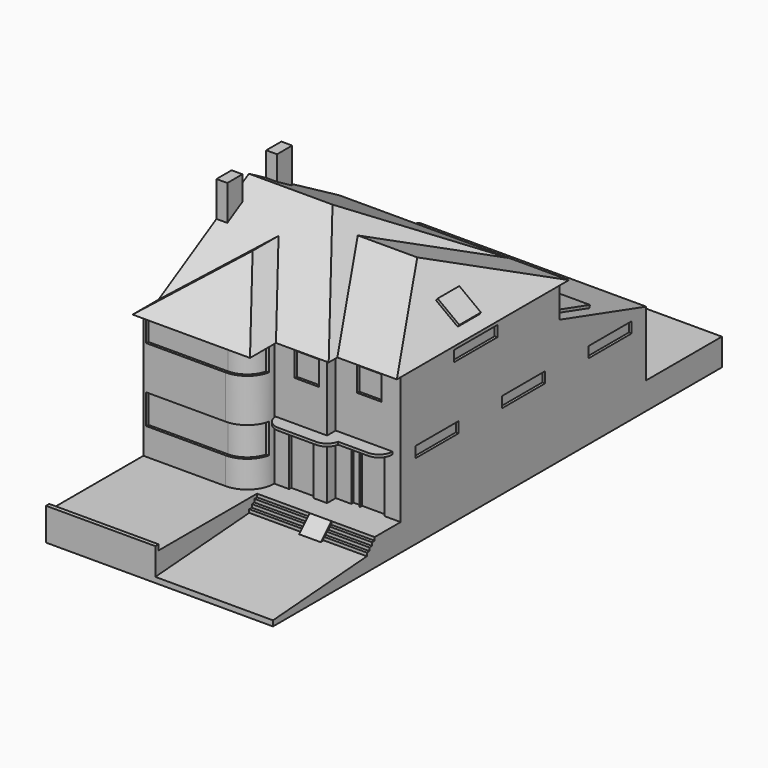
from build123d import *

# Parameters (mm, degrees)
F1_DEPTH  = 4800
F2_W      = 8392
F2_H      = 4000
F3_DEPTH  = 2400
F5_DEPTH  = 8392
F7_DEPTH  = 5992
F8_DEPTH  = 300
F11_DEPTH = 12755.001
F14_DEPTH = 500
F16_DEPTH = 8392.001
F18_DEPTH = 100
F20_DEPTH = 12755.001
F21_W     = 2000
F21_H     = 400
F22_DEPTH = 100
F23_W     = 900
F23_H     = 900
F23_H_2   = 2000
F23_W_2   = 300
F24_DEPTH = 100
F25_W     = 900
F25_H     = 2000
F25_H_2   = 900
F26_DEPTH = 100
F29_DEPTH = 1100
F32_DEPTH = 900
F34_DEPTH = 100
F36_DEPTH = 400
F37_R     = 499.99999
F38_W     = 1900
F38_H     = 2300
F39_DEPTH = 2000
F40_W     = 1238
F40_H     = 2000
F40_H_2   = 1000
F41_DEPTH = 100
F42_W     = 1200
F42_H     = 1484.5474734546
F43_DEPTH = 100
F44_W     = 1000
F44_H     = 1000
F45_DEPTH = 100
F46_W     = 671.4527505016
F46_H     = 900
F46_W_2   = 1200
F47_DEPTH = 100
F48_W     = 8392
F48_H     = 20755
F49_DEPTH = 1000
F51_DEPTH = 4350
F52_W     = 4042
F52_H     = 200
F53_DEPTH = 150
F55_DEPTH = 800


# Not quite as in the source:
# - a fillet or chamfer is up to 0.001 mm smaller than in the source, because OpenCascade refuses the exact size


with BuildPart() as f1:
    # F0 (on Top) → F1 (new body)
    with BuildSketch(Plane.XY):
        with BuildLine():
            Line((0, 11355), (0, -1400))
            Line((0, -1400), (3042, -1400))
            ThreePointArc((3042, -1400), (3749.1067811865, -1107.1067811865), (4042, -400))
            Line((4042, -400), (5992, -400))
            Line((5992, -400), (5992, 0))
            Line((5992, 0), (8392, 0))
            Line((8392, 0), (8392, 11355))
            Line((8392, 11355), (0, 11355))
        make_face()
    extrude(amount=F1_DEPTH)

    # F2 (on face) → F3 (cut)
    with BuildSketch(Plane.XY.offset(4800)):
        with Locations((4196, 9355)):
            Rectangle(F2_W, F2_H)
    extrude(amount=-F3_DEPTH, mode=Mode.SUBTRACT)

    # F4 (on face) → F5 (join, through all)
    with BuildSketch(Plane.YZ.offset(8392)):
        Polygon((7355, 2400), (11355, 2400), (7355, 3600), align=None)
    extrude(amount=-F5_DEPTH)

    # F6 (on face) → F7 (join, through all)
    with BuildSketch(Plane.YZ.offset(5992)):
        Polygon((3477.5, 7200), (-700, 4800), (-400, 4800), (0, 4800), (7655, 4800), align=None)
    extrude(amount=-F7_DEPTH)

    # F6 (on face) → F8 (join)
    with BuildSketch(Plane.YZ.offset(5992)):
        Polygon((3477.5, 7200), (-700, 4800), (7655, 4800), align=None)
    extrude(amount=F8_DEPTH)

    # F10 (on face) → F11 (cut, through all)
    with BuildSketch(Plane.XZ.offset(1400)):
        Polygon((2292, 7800), (6292, 4800), (6292, 7800), align=None)
    extrude(amount=-F11_DEPTH, mode=Mode.SUBTRACT)

    # F12 (on face) → F13 (join, up to the next surface of F1)
    with BuildSketch(Plane.XZ.offset(1400)):
        Polygon((2171, 6428.25), (0, 4800), (3042, 4800), (4342, 4800), align=None)
    extrude(until=Until.NEXT, dir=(0, 1, 0))

    # F12 (on face) → F14 (join)
    with BuildSketch(Plane.XZ.offset(1400)):
        Polygon((2171, 6428.25), (0, 4800), (4342, 4800), align=None)
    extrude(amount=F14_DEPTH)

    # F15 (on face) → F16 (cut, through all)
    with BuildSketch(Plane(origin=(0, 0, 0), x_dir=(0, -1, 0), z_dir=(-1, 0, 0))):
        Polygon((-934.17265625, 6428.25), (1900, 4800), (1900, 6428.25), align=None)
    extrude(amount=-F16_DEPTH, mode=Mode.SUBTRACT)

    # F9 (on face) → F17 (join, up to the next surface of F1)
    with BuildSketch(Plane.YZ.offset(8392)):
        Polygon((3477.5, 6500), (-300, 4800), (0, 4800), (7355, 4800), (7655, 4800), align=None)
    extrude(until=Until.NEXT, dir=(-1, 0, 0))

    # F9 (on face) → F18 (join)
    with BuildSketch(Plane.YZ.offset(8392)):
        Polygon((3477.5, 6500), (-300, 4800), (7655, 4800), align=None)
    extrude(amount=F18_DEPTH)

    # F19 (on face) → F20 (cut, through all)
    with BuildSketch(Plane.XZ.offset(1400)):
        Polygon((6225.3333333333, 6500), (8492, 4800), (8492, 6500), align=None)
    extrude(amount=-F20_DEPTH, mode=Mode.SUBTRACT)

    # F21 (on face) → F22 (cut)
    with BuildSketch(Plane.YZ.offset(8392)):
        with Locations((5677.5, 2000)):
            Rectangle(F21_W, F21_H)
        with Locations((1677.5, 2000)):
            Rectangle(F21_W, F21_H)
        with Locations((3477.5, 4400)):
            Rectangle(F21_W, F21_H)
        with Locations((9677.5, 2000)):
            Rectangle(F21_W, F21_H)
    extrude(amount=-F22_DEPTH, mode=Mode.SUBTRACT)

    # F23 (on face) → F24 (cut)
    with BuildSketch(Plane.XZ):
        with Locations((7233.0629348755, 4134.8165988922)):
            Rectangle(F23_W, F23_H)
        with Locations((7342, 1000)):
            Rectangle(F23_W, F23_H_2)
        with Locations((6722, 1000)):
            Rectangle(F23_W_2, F23_H_2)
    extrude(amount=-F24_DEPTH, mode=Mode.SUBTRACT)

    # F25 (on face) → F26 (cut)
    with BuildSketch(Plane.XZ.offset(400)):
        with Locations((5042, 1000)):
            Rectangle(F25_W, F25_H)
        with Locations((5242, 4134.8165988922)):
            Rectangle(F25_W, F25_H_2)
    extrude(amount=-F26_DEPTH, mode=Mode.SUBTRACT)

    # F28 (on offset) → F29 (cut)
    with BuildSketch(Plane(origin=(0, 0, 1000), x_dir=(1, 0, 0), z_dir=(0, 0, -1))):
        with BuildLine():
            Line((3042, 1400), (100, 1400))
            Line((100, 1400), (100, 1300))
            Line((100, 1300), (3042, 1300))
            ThreePointArc((3042, 1300), (3593.1410747417, 1111.5079168446), (3913.4249732822, 624.9855905167))
            Line((3913.4249732822, 624.9855905167), (4016.3620908368, 624.9855905167))
            ThreePointArc((4016.3620908368, 624.9855905167), (3664.5007668603, 1182.6191891708), (3042, 1400))
        make_face()
    extrude(amount=-F29_DEPTH, mode=Mode.SUBTRACT)

    # F31 (on offset) → F32 (cut)
    with BuildSketch(Plane(origin=(0, 0, 3700), x_dir=(1, 0, 0), z_dir=(0, 0, -1))):
        with BuildLine():
            Line((100, 1400), (100, 1300))
            Line((100, 1300), (3042, 1300))
            ThreePointArc((3042, 1300), (3593.1410747417, 1111.5079168446), (3913.4249732822, 624.9855905167))
            Line((3913.4249732822, 624.9855905167), (4016.3620908368, 624.9855905167))
            ThreePointArc((4016.3620908368, 624.9855905167), (3664.5007668603, 1182.6191891708), (3042, 1400))
            Line((3042, 1400), (100, 1400))
        make_face()
    extrude(amount=-F32_DEPTH, mode=Mode.SUBTRACT)

    # F33 (on face) → F34 (join)
    with BuildSketch(Plane(origin=(0, 0, 2100), x_dir=(1, 0, 0), z_dir=(0, 0, -1))):
        with BuildLine():
            Line((8092, 0), (8092, 500))
            Line((8092, 500), (6481.8979485566, 500))
            ThreePointArc((6481.8979485566, 500), (6308.2277660168, 787.2983346207), (5992, 900))
            Line((5992, 900), (4092, 900))
            Line((4092, 900), (4092, 400))
            Line((4092, 400), (5992, 400))
            Line((5992, 400), (5992, 0))
            Line((5992, 0), (8092, 0))
        make_face()
    extrude(amount=-F34_DEPTH)

    # F35 (on face) → F36 (join)
    with BuildSketch(Plane(origin=(0, 0, 0), x_dir=(0, -1, 0), z_dir=(-1, 0, 0))):
        Polygon((-2677.5, 6740.39497307), (-1977.5, 6338.2405745063), (-1977.5, 7638.2405745063), (-2677.5, 7638.2405745063), align=None)
        Polygon((-4977.5, 6338.2405745063), (-4277.5, 6740.39497307), (-4277.5, 7638.2405745063), (-4977.5, 7638.2405745063), align=None)
    extrude(amount=-F36_DEPTH)

    # F37 (radius 500 in the source; OpenCascade refuses exactly that, so slightly less here)
    f37_edges = [f1.edges().sort_by_distance(p)[0] for p in [
        (8092, -500, 2150),
        (4092, -900, 2150),
    ]]
    fillet(f37_edges, radius=F37_R)

    # F38 (on face) → F39 (cut)
    with BuildSketch(Plane(origin=(0, 11355, 0), x_dir=(-1, 0, 0), z_dir=(0, 1, 0))):
        with Locations((-7202, 1150)):
            Rectangle(F38_W, F38_H)
    extrude(amount=-F39_DEPTH, mode=Mode.SUBTRACT)

    # F40 (on face) → F41 (cut)
    with BuildSketch(Plane(origin=(0, 11355, 0), x_dir=(-1, 0, 0), z_dir=(0, 1, 0))):
        with Locations((-1469, 1000)):
            Rectangle(F40_W, F40_H)
        with Locations((-2757, 1000)):
            Rectangle(F40_W, F40_H)
        with Locations((-4045, 1000)):
            Rectangle(F40_W, F40_H)
        with Locations((-5333, 1500)):
            Rectangle(F40_W, F40_H_2)
    extrude(amount=-F41_DEPTH, mode=Mode.SUBTRACT)

    # F42 (on face) → F43 (join)
    with BuildSketch(Plane(origin=(0, 1598.119266055, 5327.0642201835), x_dir=(1, 0, 0), z_dir=(0, 0.2873478856, 0.9578262852))):
        with Locations((7292, 7352.63367649)):
            Rectangle(F42_W, F42_H)
        with Locations((1100, 7352.63367649)):
            Rectangle(F42_W, F42_H)
        with Locations((4100, 7352.63367649)):
            Rectangle(F42_W, F42_H)
    extrude(amount=F43_DEPTH)

    # F44 (on face) → F45 (join)
    with BuildSketch(Plane(origin=(5361.12, 0, 7148.16), x_dir=(0.8, 0, -0.6), z_dir=(0.6, 0, 0.8))):
        with Locations((2963.6, 3464.0258550644)):
            Rectangle(F44_W, F44_H)
    extrude(amount=F45_DEPTH)

    # F46 (on face) → F47 (cut)
    with BuildSketch(Plane(origin=(0, 7355, 0), x_dir=(-1, 0, 0), z_dir=(0, 1, 0))):
        with Locations((-5607.1791257524, 4182.3805087188)):
            Rectangle(F46_W, F46_H)
        with Locations((-4135.7263752508, 4182.3805087188)):
            Rectangle(F46_W, F46_H)
        with Locations((-1200, 4250)):
            Rectangle(F46_W_2, F46_H)
    extrude(amount=-F47_DEPTH, mode=Mode.SUBTRACT)

    # F48 (on face) → F49 (join)
    with BuildSketch(Plane(origin=(0, 0, 0), x_dir=(1, 0, 0), z_dir=(0, 0, -1))):
        with Locations((4196, -4477.5)):
            Rectangle(F48_W, F48_H)
    extrude(amount=F49_DEPTH)

    # F50 (on face) → F51 (cut, through all)
    with BuildSketch(Plane.YZ.offset(8392)):
        Polygon((-1200, -120), (-1200, 0), (-5900, 0), (-5900, -800), (-1560, -480), (-1560, -360), (-1440, -360), (-1440, -240), (-1320, -240), (-1320, -120), align=None)
    extrude(amount=-F51_DEPTH, mode=Mode.SUBTRACT)

    # F52 (on face) → F53 (join)
    with BuildSketch(Plane.XZ.offset(5900)):
        with Locations((2021, 100)):
            Rectangle(F52_W, F52_H)
    extrude(amount=-F53_DEPTH)

    # F54 (on face) → F55 (join)
    with BuildSketch(Plane.YZ.offset(5992)):
        Polygon((-1200, -489.552238806), (-1200, 0), (-1689.552238806, -489.552238806), align=None)
    extrude(amount=F55_DEPTH)


solid = f1.part
